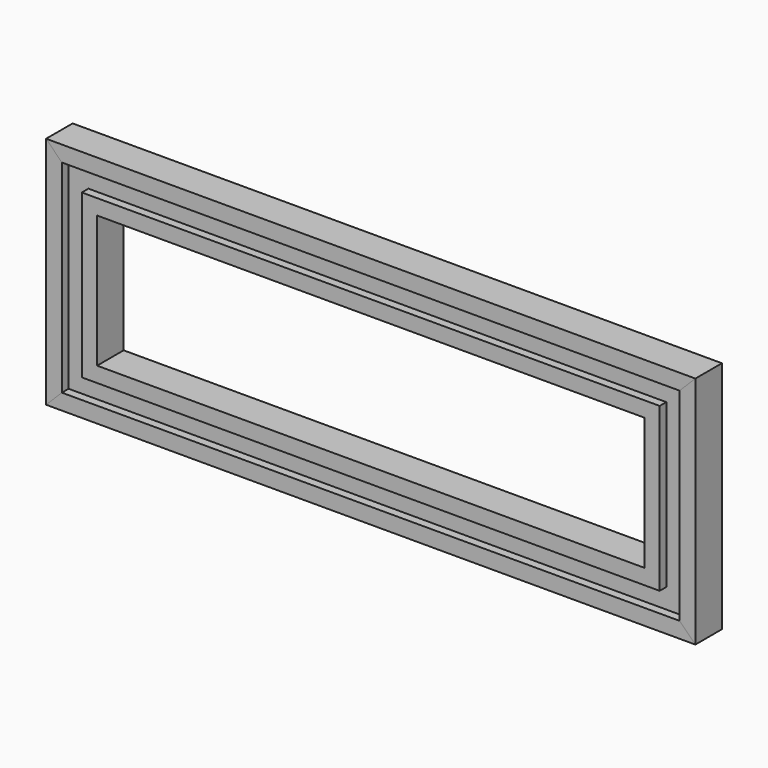
from build123d import *

# Parameters (mm, degrees)
F4_D     = 11.1125
F4_DEPTH = 12.7011486273


# Not quite as in the source:
# - a length typed as a fraction of an inch, garbled in the dataset ("3 / 203.2 mm" for 3/8 in), is restored


with BuildPart() as f2:
    # F2: sweep along a path in F1
    with BuildLine(Plane.XZ) as f2_path:
        Line((235.9086840398, 0), (0, 0))
        Line((0, 0), (-221.2913159602, 0))
        Line((-221.2913159602, 0), (-221.2913159602, 139.7))
        Line((-221.2913159602, 139.7), (235.9086840398, 139.7))
        Line((235.9086840398, 139.7), (235.9086840398, 0))
    # F0 (on Right) → F2 (sweep)
    with BuildSketch(Plane.YZ):
        Polygon((-6.35, 7.5911765571), (-6.35, -7.5911765571), (-12.7001486273, -7.648065583), (-12.6998513727, -19.7300187742), (12.7001486273, -19.7165756275), (12.6998513727, -7.6346224362), (6.35, -7.5911765571), (6.35, 7.5911765571), (12.7, 7.5911765571), (12.7, 19.2955805858), (-12.7, 19.2955805858), (-12.7, 7.5911765571), align=None)
    sweep(path=f2_path.line, transition=Transition.RIGHT)

    # F4 (through all, one way)
    with BuildSketch(Plane.XZ):
        with Locations((-220.1733291149, 139.0449106693), (-220.1733291149, 0), (0, 139.0449106693), (0, 0), (234.9551618099, 139.0449106693), (234.9551618099, 0)):
            Circle(F4_D / 2)
    extrude(amount=-F4_DEPTH, mode=Mode.SUBTRACT)


solid = f2.part
